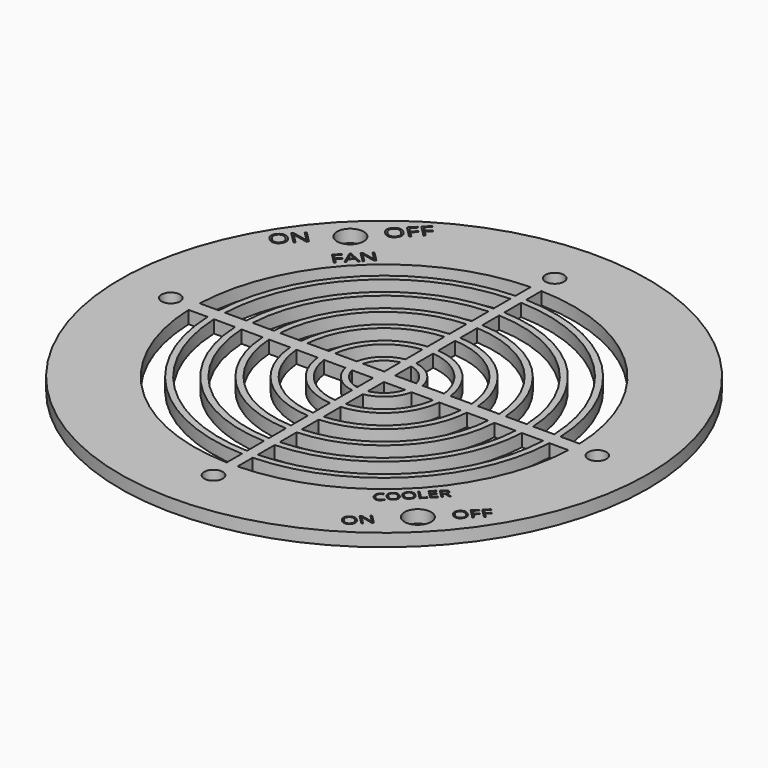
from build123d import *

# Parameters (mm, degrees)
F0_R           = 62.5
F1_DEPTH       = 3
F2_D           = 6.3
F2_DEPTH       = 50
F2_TIP         = 1.8927109499
F3_D           = 4.4
F3_DEPTH       = 50
F3_TIP         = 1.3218933619
F4_TEXT_SIZE   = 5.2055602686
F4_TEXT_SIZE_2 = 4.6449325358
F4_TEXT_SIZE_3 = 3.768532123
F4_TEXT_SIZE_4 = 4.2067271554
F5_DEPTH       = 1


# Not quite as in the source:
# - Text() gives the source's letters only with a copy of the font that has no kerning and outlines rounded to 1/6400 em; it was checked with that copy


with BuildPart() as f1:
    # F0 (on Top) → F1 (new body)
    with BuildSketch(Plane.XY):
        Circle(F0_R)
        with BuildLine():
            ThreePointArc((-1.2751998147, -44.9819282094), (-31.6849547388, -31.9540864868), (-44.969533721, -1.6556077171))
            Line((-44.969533721, -1.6556077171), (-40.4661458887, -1.6556077171))
            ThreePointArc((-40.4661458887, -1.6556077171), (-28.5029257707, -28.7720910347), (-1.2751998147, -40.4799192864))
            Line((-1.2751998147, -40.4799192864), (-1.2751998147, -44.9819282094))
        make_face(mode=Mode.SUBTRACT)
        with BuildLine():
            Line((-38.9648426545, -1.6556077171), (-33.9596667105, -1.6556077171))
            ThreePointArc((-33.9596667105, -1.6556077171), (-23.9066340586, -24.1758732621), (-1.2751998147, -33.9760778406))
            Line((-1.2751998147, -33.9760778406), (-1.2751998147, -38.9791465457))
            ThreePointArc((-1.2751998147, -38.9791465457), (-27.4422464852, -27.7114255831), (-38.9648426545, -1.6556077171))
        make_face(mode=Mode.SUBTRACT)
        with BuildLine():
            Line((-32.4578028074, -1.6556077171), (-27.4501177245, -1.6556077171))
            ThreePointArc((-27.4501177245, -1.6556077171), (-19.310284164, -19.5796559087), (-1.2751998147, -27.4704180061))
            Line((-1.2751998147, -27.4704180061), (-1.2751998147, -32.4749729089))
            ThreePointArc((-1.2751998147, -32.4749729089), (-22.8459445894, -23.1152074578), (-32.4578028074, -1.6556077171))
        make_face(mode=Mode.SUBTRACT)
        with BuildLine():
            Line((-25.9472342088, -1.6556077171), (-20.9346354897, -1.6556077171))
            ThreePointArc((-20.9346354897, -1.6556077171), (-14.7138071452, -14.9834535169), (-1.2751998147, -20.9612467528))
            Line((-1.2751998147, -20.9612467528), (-1.2751998147, -25.9687093525))
            ThreePointArc((-1.2751998147, -25.9687093525), (-18.2495741409, -18.5189914325), (-25.9472342088, -1.6556077171))
        make_face(mode=Mode.SUBTRACT)
        with BuildLine():
            Line((-19.4295898847, -1.6556077171), (-14.4051714008, -1.6556077171))
            ThreePointArc((-14.4051714008, -1.6556077171), (-10.1169702999, -10.3873438352), (-1.2751998147, -14.4438175505))
            Line((-1.2751998147, -14.4438175505), (-1.2751998147, -19.4582595684))
            ThreePointArc((-1.2751998147, -19.4582595684), (-13.6530466329, -13.9227984845), (-19.4295898847, -1.6556077171))
        make_face(mode=Mode.SUBTRACT)
        with BuildLine():
            Line((-12.8941445272, -1.6556077171), (-7.8268105309, -1.6556077171))
            ThreePointArc((-7.8268105309, -1.6556077171), (-5.5183889539, -5.7920103033), (-1.2751998147, -7.8977126709))
            Line((-1.2751998147, -7.8977126709), (-1.2751998147, -12.9373051843))
            ThreePointArc((-1.2751998147, -12.9373051843), (-9.0560341323, -9.3267489403), (-12.8941445272, -1.6556077171))
        make_face(mode=Mode.SUBTRACT)
        with BuildLine():
            ThreePointArc((-1.2751998147, -6.3736853886), (-4.4560685079, -4.7321721707), (-6.2856155695, -1.6556077171))
            Line((-6.2856155695, -1.6556077171), (-1.2751998147, -1.6556077171))
            Line((-1.2751998147, -1.6556077171), (-1.2751998147, -6.3736853886))
        make_face(mode=Mode.SUBTRACT)
        with BuildLine():
            ThreePointArc((1.2751998147, -40.4799192864), (28.5029257707, -28.7720910347), (40.4661458887, -1.6556077171))
            Line((40.4661458887, -1.6556077171), (44.969533721, -1.6556077171))
            ThreePointArc((44.969533721, -1.6556077171), (31.6849547388, -31.9540864868), (1.2751998147, -44.9819282094))
            Line((1.2751998147, -44.9819282094), (1.2751998147, -40.4799192864))
        make_face(mode=Mode.SUBTRACT)
        with BuildLine():
            ThreePointArc((1.2751998147, -33.9760778406), (23.9066340586, -24.1758732621), (33.9596667105, -1.6556077171))
            Line((33.9596667105, -1.6556077171), (38.9648426545, -1.6556077171))
            ThreePointArc((38.9648426545, -1.6556077171), (27.4422464852, -27.7114255831), (1.2751998147, -38.9791465457))
            Line((1.2751998147, -38.9791465457), (1.2751998147, -33.9760778406))
        make_face(mode=Mode.SUBTRACT)
        with BuildLine():
            ThreePointArc((1.2751998147, -27.4704180061), (19.310284164, -19.5796559087), (27.4501177245, -1.6556077171))
            Line((27.4501177245, -1.6556077171), (32.4578028074, -1.6556077171))
            ThreePointArc((32.4578028074, -1.6556077171), (22.8459445894, -23.1152074578), (1.2751998147, -32.4749729089))
            Line((1.2751998147, -32.4749729089), (1.2751998147, -27.4704180061))
        make_face(mode=Mode.SUBTRACT)
        with BuildLine():
            ThreePointArc((1.2751998147, -20.9612467528), (14.7138071452, -14.9834535169), (20.9346354897, -1.6556077171))
            Line((20.9346354897, -1.6556077171), (25.9472342088, -1.6556077171))
            ThreePointArc((25.9472342088, -1.6556077171), (18.2495741409, -18.5189914325), (1.2751998147, -25.9687093525))
            Line((1.2751998147, -25.9687093525), (1.2751998147, -20.9612467528))
        make_face(mode=Mode.SUBTRACT)
        with BuildLine():
            ThreePointArc((1.2751998147, -14.4438175505), (10.1169702999, -10.3873438352), (14.4051714008, -1.6556077171))
            Line((14.4051714008, -1.6556077171), (19.4295898847, -1.6556077171))
            ThreePointArc((19.4295898847, -1.6556077171), (13.6530466329, -13.9227984845), (1.2751998147, -19.4582595684))
            Line((1.2751998147, -19.4582595684), (1.2751998147, -14.4438175505))
        make_face(mode=Mode.SUBTRACT)
        with BuildLine():
            Line((1.2751998147, -6.3736853886), (1.2751998147, -1.6556077171))
            Line((1.2751998147, -1.6556077171), (6.2856155695, -1.6556077171))
            ThreePointArc((6.2856155695, -1.6556077171), (4.4560685079, -4.7321721707), (1.2751998147, -6.3736853886))
        make_face(mode=Mode.SUBTRACT)
        with BuildLine():
            Line((1.2751998147, -12.9373051843), (1.2751998147, -7.8977126709))
            ThreePointArc((1.2751998147, -7.8977126709), (5.5183889539, -5.7920103033), (7.8268105309, -1.6556077171))
            Line((7.8268105309, -1.6556077171), (12.8941445272, -1.6556077171))
            ThreePointArc((12.8941445272, -1.6556077171), (9.0560341323, -9.3267489403), (1.2751998147, -12.9373051843))
        make_face(mode=Mode.SUBTRACT)
        with BuildLine():
            Line((-7.8268105309, 1.6556077171), (-12.8941445272, 1.6556077171))
            ThreePointArc((-12.8941445272, 1.6556077171), (-9.0560341323, 9.3267489403), (-1.2751998147, 12.9373051843))
            Line((-1.2751998147, 12.9373051843), (-1.2751998147, 7.8977126709))
            ThreePointArc((-1.2751998147, 7.8977126709), (-5.5183889539, 5.7920103033), (-7.8268105309, 1.6556077171))
        make_face(mode=Mode.SUBTRACT)
        with BuildLine():
            Line((-1.2751998147, 1.6556077171), (-6.2856155695, 1.6556077171))
            ThreePointArc((-6.2856155695, 1.6556077171), (-4.4560685079, 4.7321721707), (-1.2751998147, 6.3736853886))
            Line((-1.2751998147, 6.3736853886), (-1.2751998147, 1.6556077171))
        make_face(mode=Mode.SUBTRACT)
        with BuildLine():
            Line((-14.4051714008, 1.6556077171), (-19.4295898847, 1.6556077171))
            ThreePointArc((-19.4295898847, 1.6556077171), (-13.6530466329, 13.9227984845), (-1.2751998147, 19.4582595684))
            Line((-1.2751998147, 19.4582595684), (-1.2751998147, 14.4438175505))
            ThreePointArc((-1.2751998147, 14.4438175505), (-10.1169702999, 10.3873438352), (-14.4051714008, 1.6556077171))
        make_face(mode=Mode.SUBTRACT)
        with BuildLine():
            Line((-20.9346354897, 1.6556077171), (-25.9472342088, 1.6556077171))
            ThreePointArc((-25.9472342088, 1.6556077171), (-18.2495741409, 18.5189914325), (-1.2751998147, 25.9687093525))
            Line((-1.2751998147, 25.9687093525), (-1.2751998147, 20.9612467528))
            ThreePointArc((-1.2751998147, 20.9612467528), (-14.7138071452, 14.9834535169), (-20.9346354897, 1.6556077171))
        make_face(mode=Mode.SUBTRACT)
        with BuildLine():
            Line((-27.4501177245, 1.6556077171), (-32.4578028074, 1.6556077171))
            ThreePointArc((-32.4578028074, 1.6556077171), (-22.8459445894, 23.1152074578), (-1.2751998147, 32.4749729089))
            Line((-1.2751998147, 32.4749729089), (-1.2751998147, 27.4704180061))
            ThreePointArc((-1.2751998147, 27.4704180061), (-19.310284164, 19.5796559087), (-27.4501177245, 1.6556077171))
        make_face(mode=Mode.SUBTRACT)
        with BuildLine():
            Line((-33.9596667105, 1.6556077171), (-38.9648426545, 1.6556077171))
            ThreePointArc((-38.9648426545, 1.6556077171), (-27.4422464852, 27.7114255831), (-1.2751998147, 38.9791465457))
            Line((-1.2751998147, 38.9791465457), (-1.2751998147, 33.9760778406))
            ThreePointArc((-1.2751998147, 33.9760778406), (-23.9066340586, 24.1758732621), (-33.9596667105, 1.6556077171))
        make_face(mode=Mode.SUBTRACT)
        with BuildLine():
            Line((-40.4661458887, 1.6556077171), (-44.969533721, 1.6556077171))
            ThreePointArc((-44.969533721, 1.6556077171), (-31.6849547388, 31.9540864868), (-1.2751998147, 44.9819282094))
            Line((-1.2751998147, 44.9819282094), (-1.2751998147, 40.4799192864))
            ThreePointArc((-1.2751998147, 40.4799192864), (-28.5029257707, 28.7720910347), (-40.4661458887, 1.6556077171))
        make_face(mode=Mode.SUBTRACT)
        with BuildLine():
            Line((6.2856155695, 1.6556077171), (1.2751998147, 1.6556077171))
            Line((1.2751998147, 1.6556077171), (1.2751998147, 6.3736853886))
            ThreePointArc((1.2751998147, 6.3736853886), (4.4560685079, 4.7321721707), (6.2856155695, 1.6556077171))
        make_face(mode=Mode.SUBTRACT)
        with BuildLine():
            Line((1.2751998147, 7.8977126709), (1.2751998147, 12.9373051843))
            ThreePointArc((1.2751998147, 12.9373051843), (9.0560341323, 9.3267489403), (12.8941445272, 1.6556077171))
            Line((12.8941445272, 1.6556077171), (7.8268105309, 1.6556077171))
            ThreePointArc((7.8268105309, 1.6556077171), (5.5183889539, 5.7920103033), (1.2751998147, 7.8977126709))
        make_face(mode=Mode.SUBTRACT)
        with BuildLine():
            Line((1.2751998147, 14.4438175505), (1.2751998147, 19.4582595684))
            ThreePointArc((1.2751998147, 19.4582595684), (13.6530466329, 13.9227984845), (19.4295898847, 1.6556077171))
            Line((19.4295898847, 1.6556077171), (14.4051714008, 1.6556077171))
            ThreePointArc((14.4051714008, 1.6556077171), (10.1169702999, 10.3873438352), (1.2751998147, 14.4438175505))
        make_face(mode=Mode.SUBTRACT)
        with BuildLine():
            Line((1.2751998147, 20.9612467528), (1.2751998147, 25.9687093525))
            ThreePointArc((1.2751998147, 25.9687093525), (18.2495741409, 18.5189914325), (25.9472342088, 1.6556077171))
            Line((25.9472342088, 1.6556077171), (20.9346354897, 1.6556077171))
            ThreePointArc((20.9346354897, 1.6556077171), (14.7138071452, 14.9834535169), (1.2751998147, 20.9612467528))
        make_face(mode=Mode.SUBTRACT)
        with BuildLine():
            Line((32.4578028074, 1.6556077171), (27.4501177245, 1.6556077171))
            ThreePointArc((27.4501177245, 1.6556077171), (19.310284164, 19.5796559087), (1.2751998147, 27.4704180061))
            Line((1.2751998147, 27.4704180061), (1.2751998147, 32.4749729089))
            ThreePointArc((1.2751998147, 32.4749729089), (22.8459445894, 23.1152074578), (32.4578028074, 1.6556077171))
        make_face(mode=Mode.SUBTRACT)
        with BuildLine():
            Line((38.9648426545, 1.6556077171), (33.9596667105, 1.6556077171))
            ThreePointArc((33.9596667105, 1.6556077171), (23.9066340586, 24.1758732621), (1.2751998147, 33.9760778406))
            Line((1.2751998147, 33.9760778406), (1.2751998147, 38.9791465457))
            ThreePointArc((1.2751998147, 38.9791465457), (27.4422464852, 27.7114255831), (38.9648426545, 1.6556077171))
        make_face(mode=Mode.SUBTRACT)
        with BuildLine():
            Line((1.2751998147, 40.4799192864), (1.2751998147, 44.9819282094))
            ThreePointArc((1.2751998147, 44.9819282094), (31.6849547388, 31.9540864868), (44.969533721, 1.6556077171))
            Line((44.969533721, 1.6556077171), (40.4661458887, 1.6556077171))
            ThreePointArc((40.4661458887, 1.6556077171), (28.5029257707, 28.7720910347), (1.2751998147, 40.4799192864))
        make_face(mode=Mode.SUBTRACT)
    extrude(amount=F1_DEPTH)

    # F2
    with Locations(Plane(origin=(0, 0, 0), x_dir=(1, 0, 0), z_dir=(0, 0, -1))):
        with Locations((-39.951533137, -39.951533137), (39.951533137, 39.951533137)):
            Hole(F2_D / 2, depth=F2_DEPTH)
            with Locations((0, 0, -(F2_DEPTH + F2_TIP / 2))):  # 118° drill point
                Cone(0, F2_D / 2, F2_TIP, mode=Mode.SUBTRACT)

    # F3
    with Locations(Plane(origin=(0, 0, 0), x_dir=(1, 0, 0), z_dir=(0, 0, -1))):
        with Locations((0, 50.5), (-50.5, 0), (50.5, 0), (0, -50.5)):
            Hole(F3_D / 2, depth=F3_DEPTH)
            with Locations((0, 0, -(F3_DEPTH + F3_TIP / 2))):  # 118° drill point
                Cone(0, F3_D / 2, F3_TIP, mode=Mode.SUBTRACT)

    # F4 (on face) → F5 (cut)
    with BuildSketch(Plane.XY.offset(3)):
        with Locations(Location((-49.9111974566, 28.3000849429), (0, 0, 45))):
            Text('ON          OFF', F4_TEXT_SIZE, font='Open Sans', text_align=(TextAlign.LEFT, TextAlign.BOTTOM))
        with Locations(Location((-36.0892031464, 29.5160734847), (0, 0, 45))):
            Text('FAN', F4_TEXT_SIZE_2, font='Open Sans', text_align=(TextAlign.LEFT, TextAlign.BOTTOM))
        with Locations(Location((29.4335613896, -39.9859406207), (0, 0, 45))):
            Text('COOLER', F4_TEXT_SIZE_3, font='Open Sans', text_align=(TextAlign.LEFT, TextAlign.BOTTOM))
        with Locations(Location((30.7792770113, -51.082375019), (0, 0, 45))):
            Text('ON             OFF', F4_TEXT_SIZE_4, font='Open Sans', text_align=(TextAlign.LEFT, TextAlign.BOTTOM))
    extrude(amount=-F5_DEPTH, mode=Mode.SUBTRACT)


solid = f1.part
